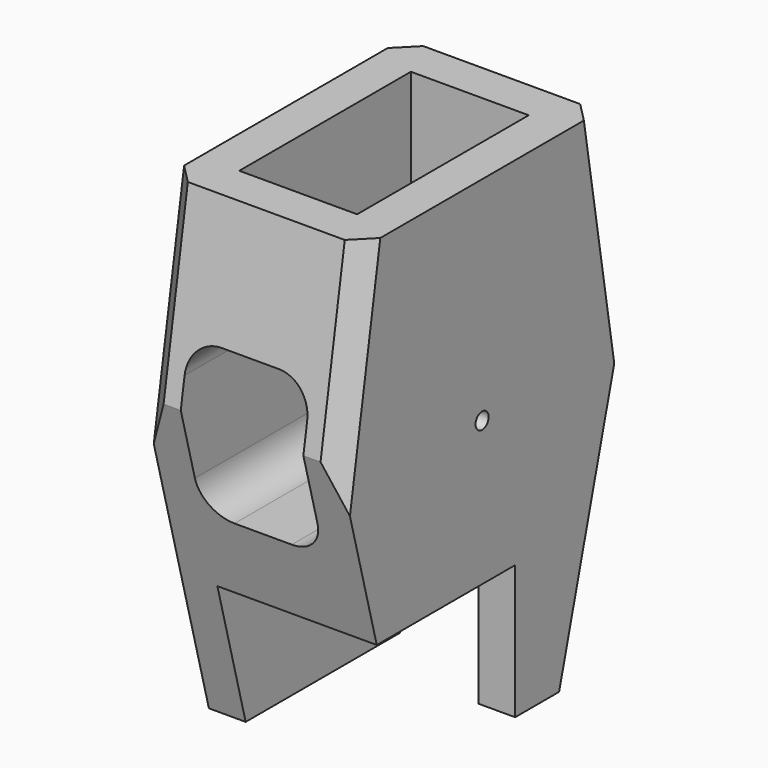
from build123d import *

# Parameters (mm, degrees)
F0_R      = 5
F1_DEPTH  = 60
F3_W      = 309.3655258417
F3_H      = 284.4564542174
F4_DEPTH  = 37.5
F5_SIZE   = 12
F7_DEPTH  = 75
F9_R      = 20
F11_DEPTH = 86.9450472691
F8_R      = 5
F7_FACE_R = 5
F12_DEPTH = 22.5


# Not quite as in the source:
# - a feature names something its author has since deleted; it is built from what else it names


with BuildPart() as f1:
    # F0 (on Right) → F1 (new body, symmetric)
    with BuildSketch(Plane.YZ):
        Polygon((75, 130), (-75, 130), (-90, 130), (-108.526711476, 17.9430459013), (-58.9007476441, -170), (58.9007476441, -170), (108.526711476, 17.9430459013), (90, 130), align=None)
        with Locations((0, -117.917008698)):
            Circle(F0_R, mode=Mode.SUBTRACT)
        Circle(F0_R, mode=Mode.SUBTRACT)
    extrude(amount=F1_DEPTH, both=True)

    # F3 (on face) → F4 (cut, symmetric)
    with BuildSketch(Plane.YZ):
        with Locations((9.2283859849, -86.6799689829)):
            Rectangle(F3_W, F3_H)
    extrude(amount=F4_DEPTH, both=True, mode=Mode.SUBTRACT)

    # F5
    f5_edges = [f1.edges().sort_by_distance(p)[0] for p in [
        (-60, -99.263356, 73.971523),
        (-60, 99.263356, 73.971523),
        (60, -99.263356, 73.971523),
        (60, 99.263356, 73.971523),
    ]]
    chamfer(f5_edges, length=F5_SIZE)

    # F6 (on face) → F7 (join, through all)
    with BuildSketch(Plane.YZ.offset(-37.5)):
        Polygon((92.4365120253, -42.9936263649), (-92.4365120253, -42.9936263649), (-80.5341079321, -88.0703141729), (80.5341079321, -88.0703141729), align=None)
    extrude(amount=F7_DEPTH)

    # F9
    f9_edges = [f1.edges().sort_by_distance(p)[0] for p in [
        (-37.5, 0, 55.548258),
        (37.5, 0, 55.548258),
        (-37.5, 0, -42.993626),
        (37.5, 0, -42.993626),
    ]]
    fillet(f9_edges, radius=F9_R)

    # F10 (on face) → F11 (cut, through all)
    with BuildSketch(Plane.XY.offset(130)):
        Polygon((36.0373817384, 65.5976682901), (0, 65.5976682901), (-36.0373817384, 65.5976682901), (-36.0373817384, 0), (-36.0373817384, -65.5976682901), (0, -65.5976682901), (36.0373817384, -65.5976682901), (36.0373817384, 0), align=None)
    extrude(amount=-F11_DEPTH, mode=Mode.SUBTRACT)

    # F8 (on face) + F7_face (on face) → F12 (cut, through all)
    with BuildSketch(Plane.YZ.offset(60)):
        Polygon((25.2734031528, -88.0703141729), (-80.5341079321, -88.0703141729), (-58.9007476441, -170), (25.2734031528, -170), align=None)
        with Locations((0, -117.917008698)):
            Circle(F8_R, mode=Mode.SUBTRACT)
    with BuildSketch(Plane(origin=(37.5, 0, -126.978888881), x_dir=(0, -1, 0), z_dir=(-1, 0, 0))):
        Polygon((-80.5341079321, 38.9085747081), (-58.9007476441, -43.021111119), (58.9007476441, -43.021111119), (80.5341079321, 38.9085747081), align=None)
        with Locations((0, 9.061880183)):
            Circle(F7_FACE_R, mode=Mode.SUBTRACT)
    extrude(amount=-F12_DEPTH, dir=(1, 0, 0), mode=Mode.SUBTRACT)


solid = f1.part
